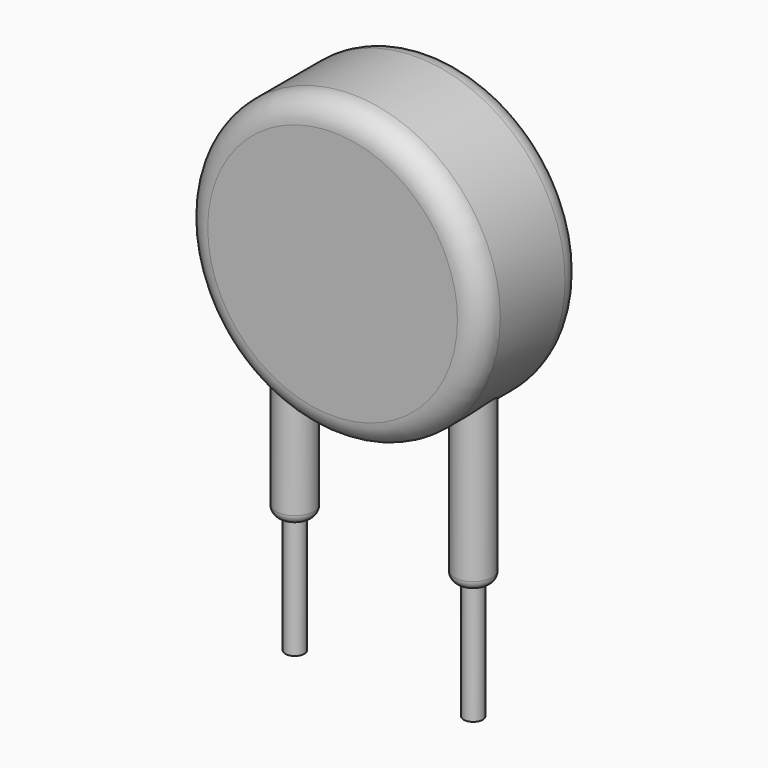
from build123d import *

# Parameters (mm, degrees)
F0_R     = 6.25
F1_DEPTH = 2.7
F2_R     = 0.8
F2_R_2   = 0.4
F4_DEPTH = 5
F5_R     = 0.39999
F6_R     = 1


# Not quite as in the source:
# - a fillet or chamfer is up to 0.001 mm smaller than in the source, because OpenCascade refuses the exact size
# - a feature names something its author has since deleted; it is built from what else it names


with BuildPart() as f1:
    # F0 (on Front) → F1 (new body, symmetric)
    with BuildSketch(Plane.XZ):
        with Locations((0, 11.25)):
            Circle(F0_R)
    extrude(amount=F1_DEPTH, both=True)

    # F2 (on Top) → F3 (join, up to the next surface of F1)
    with BuildSketch(Plane.XY):
        with Locations((-3.75, 0)):
            Circle(F2_R)
        with Locations((-3.75, 0)):
            Circle(F2_R_2, mode=Mode.SUBTRACT)
        with Locations((3.75, 0)):
            Circle(F2_R)
        with Locations((3.75, 0)):
            Circle(F2_R_2, mode=Mode.SUBTRACT)
        with Locations((-3.75, 0)):
            Circle(F2_R_2)
        with Locations((3.75, 0)):
            Circle(F2_R_2)
    extrude(until=Until.NEXT)

    # F2 (on Top) → F4 (join)
    with BuildSketch(Plane.XY):
        with Locations((-3.75, 0)):
            Circle(F2_R_2)
        with Locations((3.75, 0)):
            Circle(F2_R_2)
    extrude(amount=-F4_DEPTH)

    # F5 (radius 0.4 in the source; OpenCascade refuses exactly that, so slightly less here)
    f5_edges = [f1.edges().sort_by_distance(p)[0] for p in [
        (-4.55, 0, 0),
        (2.95, 0, 0),
    ]]
    fillet(f5_edges, radius=F5_R)

    # F6
    f6_edges = [f1.edges().sort_by_distance(p)[0] for p in [
        (-6.25, -2.7, 11.25),
        (-6.25, 2.7, 11.25),
    ]]
    fillet(f6_edges, radius=F6_R)


solid = f1.part
